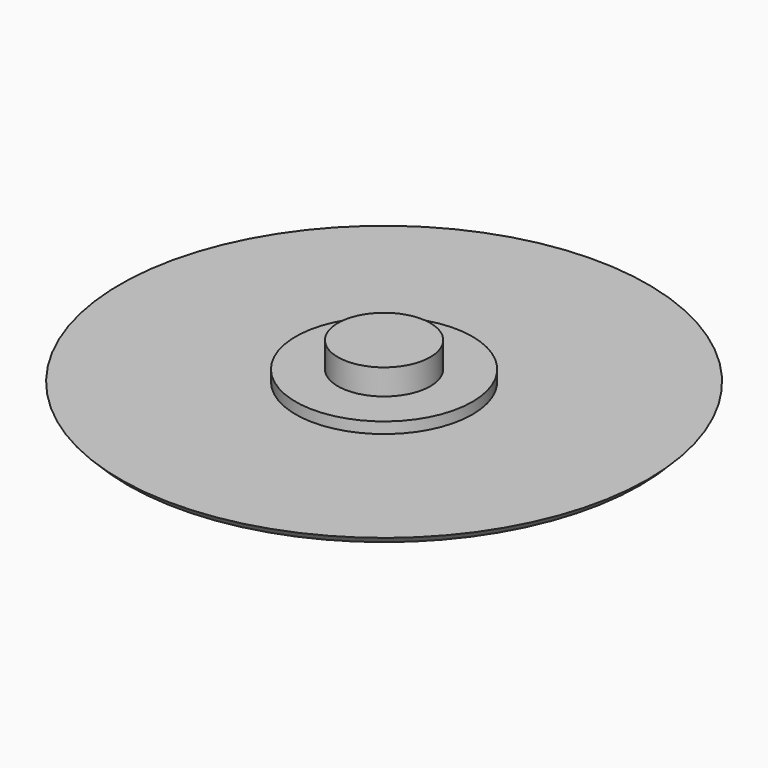
from build123d import *

# Parameters (mm, degrees)
F0_R     = 25
F0_R_2   = 7.9354206637
F1_DEPTH = 0.7
F0_R_3   = 4.15
F2_DEPTH = 1.7
F3_DEPTH = 4


# Not quite as in the source:
# - a fillet or chamfer that OpenCascade refuses, or shapes differently, is made with other operations: its cross-section is extruded or revolved along the edge and cut away or added


with BuildPart() as f1:
    # F0 (on Top) → F1 (new body)
    with BuildSketch(Plane.XY):
        Circle(F0_R)
        Circle(F0_R_2, mode=Mode.SUBTRACT)
    extrude(amount=F1_DEPTH)

    # F0 (on Top) → F2 (join)
    with BuildSketch(Plane.XY):
        Circle(F0_R_2)
        Circle(F0_R_3, mode=Mode.SUBTRACT)
    extrude(amount=F2_DEPTH)

    # F0 (on Top) → F3 (join)
    with BuildSketch(Plane.XY):
        Circle(F0_R_3)
    extrude(amount=F3_DEPTH)

    # F4: chamfer of 2 on 1 edges, made by hand

    # F4_s1 → F4_t2 (revolve, cut)
    with BuildSketch(Plane.XZ):
        Polygon((25, 2), (23, 0), (25, 0), align=None)
    revolve(axis=Axis((0, 0, 0), (0, 0, 1)), mode=Mode.SUBTRACT)


solid = f1.part
